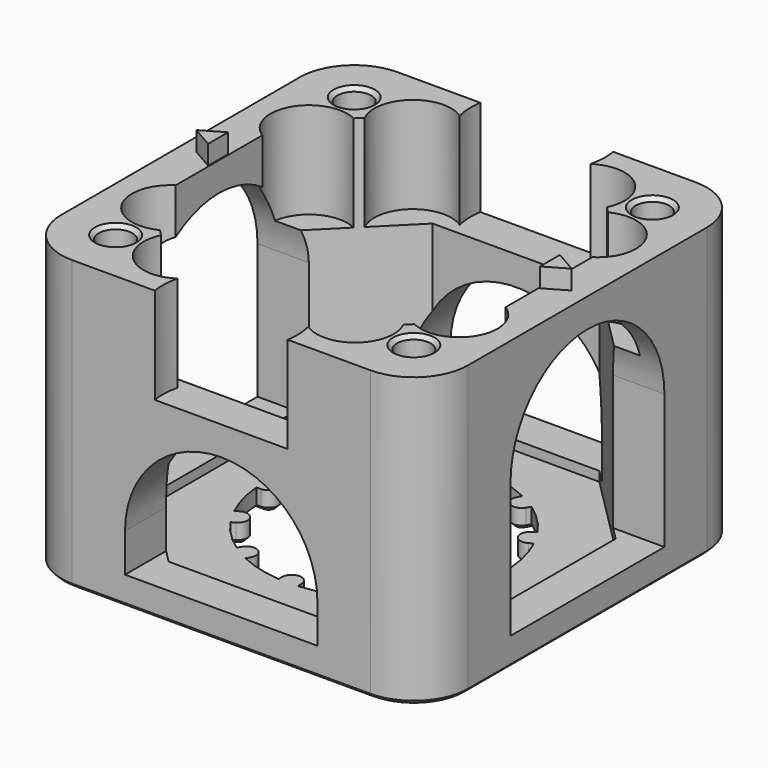
from build123d import *

# Parameters (mm, degrees)
F0_W            = 42.3
F0_H            = 42.3
F0_R            = 1.75
F0_R_2          = 12.5
F1_DEPTH        = 30
F3_DEPTH        = 30
F3_COPIES_COUNT = 12
F5_DEPTH        = 28
F6_R            = 4
F7_DEPTH        = 10
F9_DEPTH        = 2
F11_DEPTH       = 42.301
F13_DEPTH       = 42.301
F14_R           = 5.65
F15_SIZE        = 0.4


# Not quite as in the source:
# - two fillets or chamfers of one size are made in one step
# - a pattern or mirror of a feature is missing from the dataset's text; its kind, count and spacing are read off the source's solid


with BuildPart() as f1:
    # F0 (on Top) → F1 (new body)
    with BuildSketch(Plane.XY):
        Rectangle(F0_W, F0_H)
        with Locations((-15.5, -15.5)):
            Circle(F0_R, mode=Mode.SUBTRACT)
        with Locations((15.5, -15.5)):
            Circle(F0_R, mode=Mode.SUBTRACT)
        with Locations((-15.5, 15.5)):
            Circle(F0_R, mode=Mode.SUBTRACT)
        Circle(F0_R_2, mode=Mode.SUBTRACT)
        with Locations((15.5, 15.5)):
            Circle(F0_R, mode=Mode.SUBTRACT)
    extrude(amount=F1_DEPTH)

    # F2 (on Top) → F3 (join)
    with BuildSketch(Plane.XY):
        with BuildLine():
            Line((13, 1), (12, 1))
            ThreePointArc((12, 1), (11, 0), (12, -1))
            Line((12, -1), (13, -1))
            Line((13, -1), (13, 1))
        make_face()
    f3 = extrude(amount=F3_DEPTH)

    # F3_copies: F3 ×12 about axis
    f3_copies_axis = Axis((0, 0, 0), (0, 0, 1))
    for i in range(1, F3_COPIES_COUNT):
        add(f3.rotate(f3_copies_axis, i * 360 / F3_COPIES_COUNT))

    # F4 (on face) → F5 (cut)
    with BuildSketch(Plane.XY.offset(30)):
        Polygon((8.6647186258, 17.15), (-8.6647186258, 17.15), (-17.15, 8.6647186258), (-17.15, -8.6647186258), (-8.6647186258, -17.15), (8.6647186258, -17.15), (17.15, -8.6647186258), (17.15, 8.6647186258), align=None)
    extrude(amount=-F5_DEPTH, mode=Mode.SUBTRACT)

    # F6 (on face) → F7 (cut)
    with BuildSketch(Plane.XY.offset(30)):
        with BuildLine():
            ThreePointArc((-5.0013098527, -15.1023577349), (-5.0003274766, -15.0511830577), (-5, -15))
            ThreePointArc((-5, -15), (-12.5211995286, -13.1023293543), (-6.8005769398, -18.3410384916))
            ThreePointArc((-6.8005769398, -18.3410384916), (-6.1191009329, -16.6004994817), (-5.0013098527, -15.1023577349))
        make_face()
        with BuildLine():
            ThreePointArc((-5.0013098527, -15.1023577349), (-6.1191009329, -16.6004994817), (-6.8005769398, -18.3410384916))
            ThreePointArc((-6.8005769398, -18.3410384916), (-5.5033708955, -16.9425717247), (-5.0013098527, -15.1023577349))
        make_face()
        with BuildLine():
            ThreePointArc((-5.0013098527, -15.1023577349), (-5.5033708955, -16.9425717247), (-6.8005769398, -18.3410384916))
            ThreePointArc((-6.8005769398, -18.3410384916), (-0.8354523989, -26.9499654164), (7, -20))
            ThreePointArc((7, -20), (6.9499654164, -19.1645476011), (6.8005769398, -18.3410384916))
            ThreePointArc((6.8005769398, -18.3410384916), (5.5033708955, -16.9425717247), (5.0013098527, -15.1023577349))
            ThreePointArc((5.0013098527, -15.1023577349), (0, -13), (-5.0013098527, -15.1023577349))
        make_face()
        with BuildLine():
            ThreePointArc((6.8005769398, -18.3410384916), (6.1191009329, -16.6004994817), (5.0013098527, -15.1023577349))
            ThreePointArc((5.0013098527, -15.1023577349), (5.5033708955, -16.9425717247), (6.8005769398, -18.3410384916))
        make_face()
        with BuildLine():
            ThreePointArc((13, -15), (8.9488169423, -11.0003274766), (5.0013098527, -15.1023577349))
            ThreePointArc((5.0013098527, -15.1023577349), (6.1191009329, -16.6004994817), (6.8005769398, -18.3410384916))
            ThreePointArc((6.8005769398, -18.3410384916), (10.8976706457, -18.5211995286), (13, -15))
        make_face()
        with BuildLine():
            ThreePointArc((-6.8005769398, 18.3410384916), (-12.5211995286, 13.1023293543), (-5, 15))
            ThreePointArc((-5, 15), (-5.0003274766, 15.0511830577), (-5.0013098527, 15.1023577349))
            ThreePointArc((-5.0013098527, 15.1023577349), (-6.1191009329, 16.6004994817), (-6.8005769398, 18.3410384916))
        make_face()
        with BuildLine():
            ThreePointArc((-6.8005769398, 18.3410384916), (-6.1191009329, 16.6004994817), (-5.0013098527, 15.1023577349))
            ThreePointArc((-5.0013098527, 15.1023577349), (-5.5033708955, 16.9425717247), (-6.8005769398, 18.3410384916))
        make_face()
        with BuildLine():
            ThreePointArc((-6.8005769398, 18.3410384916), (-5.5033708955, 16.9425717247), (-5.0013098527, 15.1023577349))
            ThreePointArc((-5.0013098527, 15.1023577349), (0, 13), (5.0013098527, 15.1023577349))
            ThreePointArc((5.0013098527, 15.1023577349), (5.5033708955, 16.9425717247), (6.8005769398, 18.3410384916))
            ThreePointArc((6.8005769398, 18.3410384916), (6.9499654164, 19.1645476011), (7, 20))
            ThreePointArc((7, 20), (-0.8354523989, 26.9499654164), (-6.8005769398, 18.3410384916))
        make_face()
        with BuildLine():
            ThreePointArc((6.8005769398, 18.3410384916), (6.1191009329, 16.6004994817), (5.0013098527, 15.1023577349))
            ThreePointArc((5.0013098527, 15.1023577349), (8.9488169423, 11.0003274766), (13, 15))
            ThreePointArc((13, 15), (10.8976706457, 18.5211995286), (6.8005769398, 18.3410384916))
        make_face()
        with BuildLine():
            ThreePointArc((6.8005769398, 18.3410384916), (5.5033708955, 16.9425717247), (5.0013098527, 15.1023577349))
            ThreePointArc((5.0013098527, 15.1023577349), (6.1191009329, 16.6004994817), (6.8005769398, 18.3410384916))
        make_face()
        with Locations((-15, -9)):
            Circle(F6_R)
        with Locations((-15, 9)):
            Circle(F6_R)
        with Locations((15, 9)):
            Circle(F6_R)
        with Locations((15, -9)):
            Circle(F6_R)
    extrude(amount=-F7_DEPTH, mode=Mode.SUBTRACT)

    # F8 (on face) → F9 (join)
    with BuildSketch(Plane.XY.offset(30)):
        Polygon((-19.5, 0), (-17.25, -1.2990381057), (-17.25, 1.2990381057), align=None)
        Polygon((19.4999994221, 0.0013167423), (17.2488599567, 1.298379234), (17.2511406212, -1.2996959763), align=None)
    extrude(amount=F9_DEPTH)

    # F10 (on face) → F11 (cut, through all)
    with BuildSketch(Plane.XZ.offset(21.15)):
        with BuildLine():
            ThreePointArc((10, 7), (0, 17), (-10, 7))
            Line((-10, 7), (-10, 3))
            Line((-10, 3), (10, 3))
            Line((10, 3), (10, 7))
        make_face()
    extrude(amount=-F11_DEPTH, mode=Mode.SUBTRACT)

    # F12 (on face) → F13 (cut, through all)
    with BuildSketch(Plane.YZ.offset(21.15)):
        with BuildLine():
            ThreePointArc((10, 17), (0, 27), (-10, 17))
            Line((-10, 17), (-10, 3))
            Line((-10, 3), (10, 3))
            Line((10, 3), (10, 17))
        make_face()
    extrude(amount=-F13_DEPTH, mode=Mode.SUBTRACT)

    # F14
    f14_edges = [f1.edges().sort_by_distance(p)[0] for p in [
        (21.15, -21.15, 15),
        (21.15, 21.15, 15),
        (-21.15, -21.15, 15),
        (-21.15, 21.15, 15),
    ]]
    fillet(f14_edges, radius=F14_R)

    # F15
    f15_edges = [f1.edges().sort_by_distance(p)[0] for p in [
        (-21.15, 0, 0),
        (-19.495153, 19.495153, 0),
        (-19.495153, -19.495153, 0),
        (0, 21.15, 0),
        (0, -21.15, 0),
        (19.495153, 19.495153, 0),
        (19.495153, -19.495153, 0),
        (21.15, 0, 0),
        (-17.25, -15.5, 0),
        (13.75, -15.5, 0),
        (-17.25, 15.5, 0),
        (12.074073, 3.235238, 0),
        (12.229968, 1, 0),
        (11, 0, 0),
        (12.229968, -1, 0),
        (12.074073, -3.235238, 0),
        (11.091463, -5.248959, 0),
        (9.526279, -5.5, 0),
        (10.091463, -6.981009, 0),
        (8.838835, -8.838835, 0),
        (6.981009, -10.091463, 0),
        (5.5, -9.526279, 0),
        (5.248959, -11.091463, 0),
        (3.235238, -12.074073, 0),
        (1, -12.229968, 0),
        (0, -11, 0),
        (-1, -12.229968, 0),
        (-3.235238, -12.074073, 0),
        (-5.248959, -11.091463, 0),
        (-5.5, -9.526279, 0),
        (-6.981009, -10.091463, 0),
        (-8.838835, -8.838835, 0),
        (-10.091463, -6.981009, 0),
        (-9.526279, -5.5, 0),
        (-11.091463, -5.248959, 0),
        (-12.074073, -3.235238, 0),
        (-12.229968, -1, 0),
        (-11, 0, 0),
        (-12.229968, 1, 0),
        (-12.074073, 3.235238, 0),
        (-11.091463, 5.248959, 0),
        (-9.526279, 5.5, 0),
        (-10.091463, 6.981009, 0),
        (-8.838835, 8.838835, 0),
        (-6.981009, 10.091463, 0),
        (-5.5, 9.526279, 0),
        (-5.248959, 11.091463, 0),
        (-3.235238, 12.074073, 0),
        (-1, 12.229968, 0),
        (0, 11, 0),
        (1, 12.229968, 0),
        (3.235238, 12.074073, 0),
        (5.248959, 11.091463, 0),
        (5.5, 9.526279, 0),
        (6.981009, 10.091463, 0),
        (8.838835, 8.838835, 0),
        (10.091463, 6.981009, 0),
        (9.526279, 5.5, 0),
        (11.091463, 5.248959, 0),
        (13.75, 15.5, 0),
        (-17.25, -15.5, 30),
        (-17.25, 15.5, 30),
        (13.75, -15.5, 30),
        (13.75, 15.5, 30),
    ]]
    chamfer(f15_edges, length=F15_SIZE)


solid = f1.part
